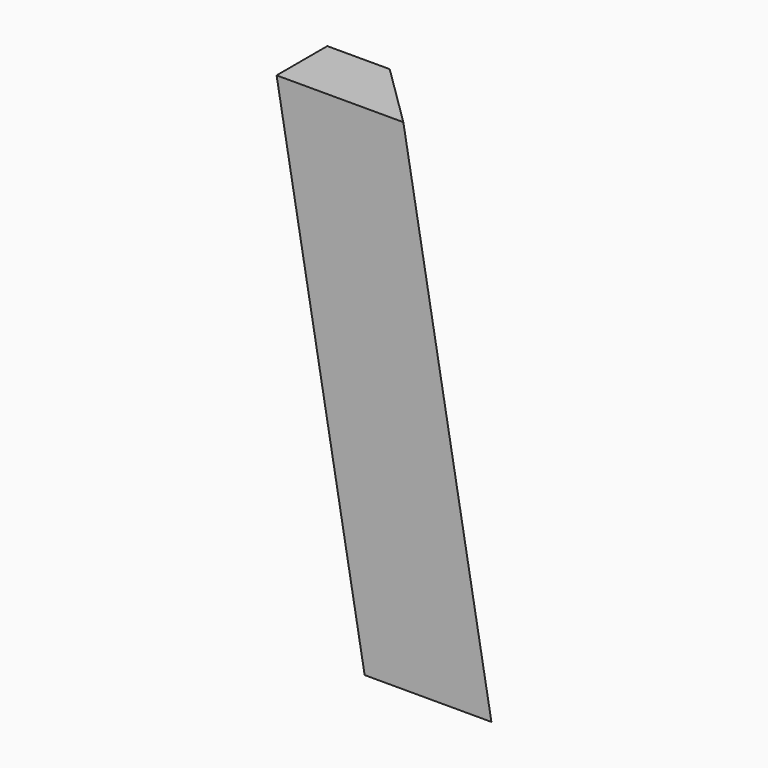
from build123d import *

# Parameters (mm, degrees)
F1_DEPTH = 20
F2_SIZE  = 19.99999


# Not quite as in the source:
# - a fillet or chamfer is up to 0.001 mm smaller than in the source, because OpenCascade refuses the exact size


with BuildPart() as f1:
    # F0 (on Front) → F1 (new body)
    with BuildSketch(Plane.XZ):
        Polygon((40, 0), (0, 0), (27.7837084267, -157.569240482), (67.7837084267, -157.569240482), align=None)
    extrude(amount=F1_DEPTH)

    # F2 (size 20 in the source; OpenCascade refuses exactly that, so slightly less here)
    f2_edges = [f1.edges().sort_by_distance(p)[0] for p in [
        (53.891854, 0, -78.78462),
    ]]
    chamfer(f2_edges, length=F2_SIZE)


solid = f1.part
